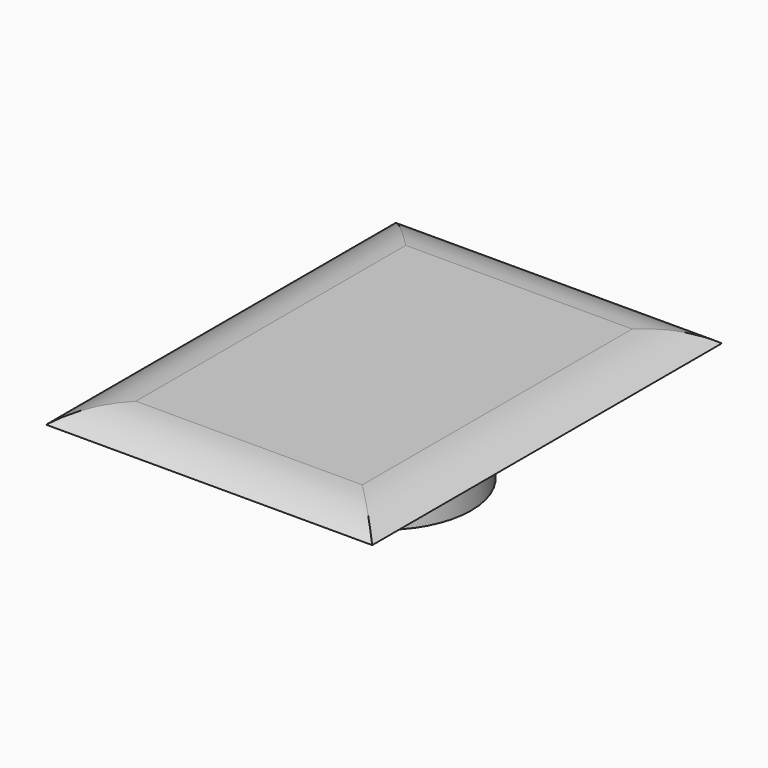
from build123d import *

# Parameters (mm, degrees)
F0_R        = 10.5
F0_R_2      = 9.5
F1_DEPTH    = 10
F2_W        = 39.2694026232
F2_H        = 52.6303946972
F3_DEPTH    = 1
F4_DEPTH    = 1
F5_T1_DEPTH = 82.6303946972
F5_T3_DEPTH = 69.2694026232


# Not quite as in the source:
# - a fillet or chamfer that OpenCascade refuses, or shapes differently, is made with other operations: its cross-section is extruded or revolved along the edge and cut away or added


with BuildPart() as f1:
    # F0 (on Top) → F1 (new body)
    with BuildSketch(Plane.XY):
        Circle(F0_R)
        Circle(F0_R_2, mode=Mode.SUBTRACT)
    extrude(amount=-F1_DEPTH)

    # F2 (on Top) → F3 (join)
    with BuildSketch(Plane.XY):
        Rectangle(F2_W, F2_H)
    extrude(amount=F3_DEPTH)

    # F4 (add): a face of the model
    f4_faces = [f1.faces().sort_by_distance(p)[0] for p in [
        (0, 0, 1),
    ]]
    extrude(f4_faces, amount=F4_DEPTH)

    # F5: fillet of radius 10 on 4 edges, made by hand

    # F5_s2 → F5_t1 (cut)
    with BuildSketch(Plane.XZ.offset(-41.3151973486)):
        with BuildLine():
            ThreePointArc((19.6347013116, 0), (16.7969789718, 1.4868329805), (13.6347013116, 2))
            Line((13.6347013116, 2), (19.6347013116, 2))
            Line((19.6347013116, 2), (19.6347013116, 0))
        make_face()
        with BuildLine():
            ThreePointArc((-19.6347013116, 0), (-16.7969789718, 1.4868329805), (-13.6347013116, 2))
            Line((-13.6347013116, 2), (-19.6347013116, 2))
            Line((-19.6347013116, 2), (-19.6347013116, 0))
        make_face()
    extrude(amount=F5_T1_DEPTH, mode=Mode.SUBTRACT)

    # F5_s4 → F5_t3 (cut)
    with BuildSketch(Plane.YZ.offset(-34.6347013116)):
        with BuildLine():
            ThreePointArc((26.3151973486, 0), (23.4774750088, 1.4868329805), (20.3151973486, 2))
            Line((20.3151973486, 2), (26.3151973486, 2))
            Line((26.3151973486, 2), (26.3151973486, 0))
        make_face()
        with BuildLine():
            ThreePointArc((-20.3151973486, 2), (-23.4774750088, 1.4868329805), (-26.3151973486, 0))
            Line((-26.3151973486, 0), (-26.3151973486, 2))
            Line((-26.3151973486, 2), (-20.3151973486, 2))
        make_face()
    extrude(amount=F5_T3_DEPTH, mode=Mode.SUBTRACT)


solid = f1.part
